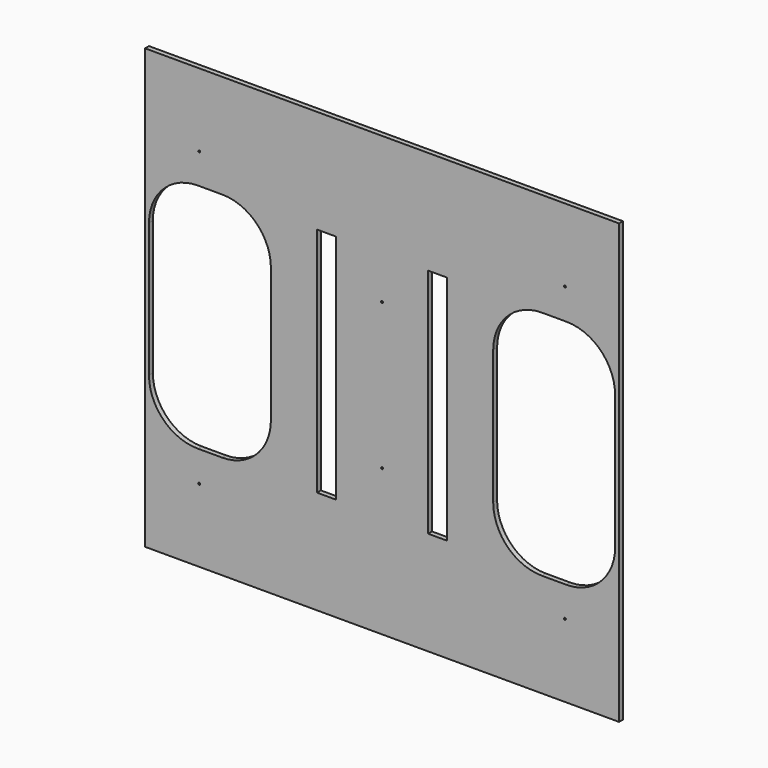
from build123d import *

# Parameters (mm, degrees)
F0_W     = 493.776
F0_H     = 457.2
F0_W_2   = 19.812
F0_H_2   = 241.3
F1_DEPTH = 5.08
F2_R     = 1.016
F3_DEPTH = 5.081
F5_DEPTH = 5.081
F6_DEPTH = 5.08


# Not quite as in the source:
# - a feature names something its author has since deleted; it is built from what else it names


with BuildPart() as f1:
    # F0 (on Front) → F1 (new body)
    with BuildSketch(Plane.XZ):
        with Locations((246.888, 228.6)):
            Rectangle(F0_W, F0_H)
        with Locations((188.9506, 228.6)):
            Rectangle(F0_W_2, F0_H_2, mode=Mode.SUBTRACT)
        with Locations((304.8254, 228.6)):
            Rectangle(F0_W_2, F0_H_2, mode=Mode.SUBTRACT)
    extrude(amount=F1_DEPTH)

    # F2 (on face) → F3 (cut, through all)
    with BuildSketch(Plane.XZ.offset(5.08)):
        with Locations((56.388, 381)):
            Circle(F2_R)
        with Locations((56.388, 76.2)):
            Circle(F2_R)
        with Locations((437.388, 76.2)):
            Circle(F2_R)
        with Locations((437.388, 381)):
            Circle(F2_R)
    extrude(amount=-F3_DEPTH, mode=Mode.SUBTRACT)

    # F4 (on face) → F5 (cut, through all)
    with BuildSketch(Plane.XZ.offset(5.08)):
        with BuildLine():
            Line((80.2894, 349.25), (54.8894, 349.25))
            ThreePointArc((54.8894, 349.25), (18.9683755157, 334.3710244843), (4.0894, 298.45))
            Line((4.0894, 298.45), (4.0894, 158.75))
            ThreePointArc((4.0894, 158.75), (18.9683755157, 122.8289755157), (54.8894, 107.95))
            Line((54.8894, 107.95), (80.2894, 107.95))
            ThreePointArc((80.2894, 107.95), (116.2104244843, 122.8289755157), (131.0894, 158.75))
            Line((131.0894, 158.75), (131.0894, 298.45))
            ThreePointArc((131.0894, 298.45), (116.2104244843, 334.3710244843), (80.2894, 349.25))
        make_face()
        with BuildLine():
            Line((438.8866, 349.25), (413.4866, 349.25))
            ThreePointArc((413.4866, 349.25), (377.5655755157, 334.3710244843), (362.6866, 298.45))
            Line((362.6866, 298.45), (362.6866, 158.75))
            ThreePointArc((362.6866, 158.75), (377.5655755157, 122.8289755157), (413.4866, 107.95))
            Line((413.4866, 107.95), (438.8866, 107.95))
            ThreePointArc((438.8866, 107.95), (474.8076244843, 122.8289755157), (489.6866, 158.75))
            Line((489.6866, 158.75), (489.6866, 298.45))
            ThreePointArc((489.6866, 298.45), (474.8076244843, 334.3710244843), (438.8866, 349.25))
        make_face()
    extrude(amount=-F5_DEPTH, mode=Mode.SUBTRACT)

    # F2 (on face) → F6 (cut, through all)
    with BuildSketch(Plane.XZ.offset(5.08)):
        with Locations((246.888, 304.8)):
            Circle(F2_R)
        with Locations((246.888, 152.4)):
            Circle(F2_R)
    extrude(amount=-F6_DEPTH, mode=Mode.SUBTRACT)


solid = f1.part
